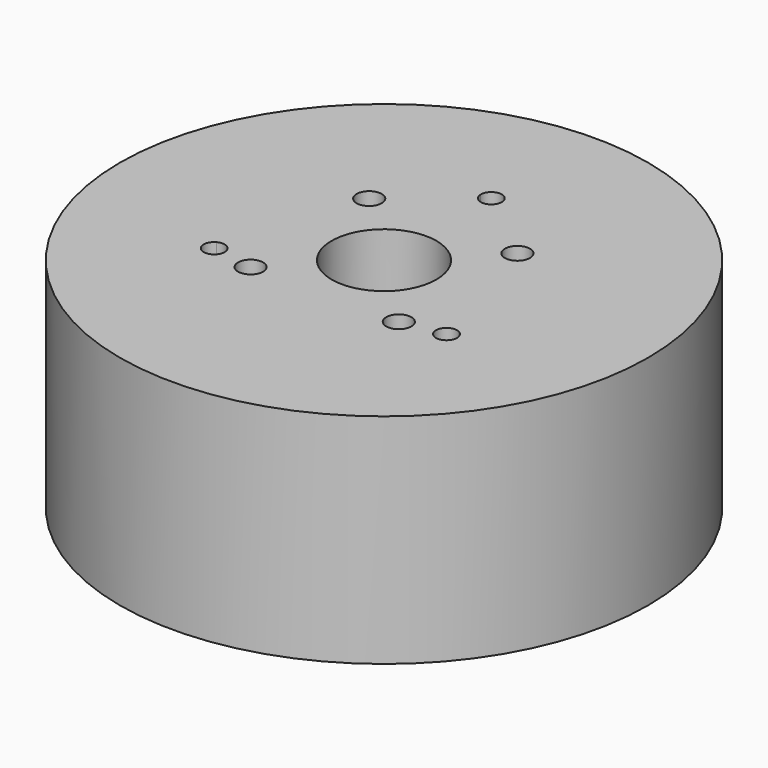
from build123d import *

# Parameters (mm, degrees)
F0_R     = 31.5
F0_R_2   = 1.5
F0_R_3   = 6.25
F1_DEPTH = 13
F2_DEPTH = 13


# Not quite as in the source:
# - a feature names something its author has since deleted; it is built from what else it names


with BuildPart() as f1:
    # F0 (on Top) → F1 (new body)
    with BuildSketch(Plane.XY):
        Circle(F0_R)
        with BuildLine():
            ThreePointArc((1.2490459616, 15.951171875), (11.7470152674, 10.8631317909), (16, 0))
            ThreePointArc((16, 0), (15.6047795357, -3.5342404619), (14.4386430447, -6.8938804043))
            ThreePointArc((14.4386430447, -6.8938804043), (14.9265222791, -7.3539720324), (15.1064064606, -8))
            ThreePointArc((15.1064064606, -8), (14.4601399606, -9.0945345408), (13.1895970831, -9.0572914707))
            ThreePointArc((13.1895970831, -9.0572914707), (0, -16), (-13.1895970831, -9.0572914707))
            ThreePointArc((-13.1895970831, -9.0572914707), (-14.9389382153, -8.625), (-14.4386430447, -6.8938804043))
            ThreePointArc((-14.4386430447, -6.8938804043), (-13.8564064606, 8), (-1.2490459616, 15.951171875))
            ThreePointArc((-1.2490459616, 15.951171875), (-0.0244187222, 17.2497614676), (1.25, 16))
            ThreePointArc((1.25, 16), (1.2497614676, 15.9755812778), (1.2490459616, 15.951171875))
        make_face(mode=Mode.SUBTRACT)
        with BuildLine():
            ThreePointArc((14.4386430447, -6.8938804043), (15.6047795357, -3.5342404619), (16, 0))
            ThreePointArc((16, 0), (11.7470152674, 10.8631317909), (1.2490459616, 15.951171875))
            ThreePointArc((1.2490459616, 15.951171875), (0, 14.75), (-1.2490459616, 15.951171875))
            ThreePointArc((-1.2490459616, 15.951171875), (-13.8564064606, 8), (-14.4386430447, -6.8938804043))
            ThreePointArc((-14.4386430447, -6.8938804043), (-13.210378493, -6.9298841815), (-12.6064064606, -8))
            ThreePointArc((-12.6064064606, -8), (-12.7618719198, -8.6037335), (-13.1895970831, -9.0572914707))
            ThreePointArc((-13.1895970831, -9.0572914707), (0, -16), (13.1895970831, -9.0572914707))
            ThreePointArc((13.1895970831, -9.0572914707), (12.7738747058, -7.375), (14.4386430447, -6.8938804043))
        make_face()
        with Locations((-8.8388347648, -8.8388347648)):
            Circle(F0_R_2, mode=Mode.SUBTRACT)
        with Locations((8.8388347648, -8.8388347648)):
            Circle(F0_R_2, mode=Mode.SUBTRACT)
        with Locations((-8.8388347648, 8.8388347648)):
            Circle(F0_R_2, mode=Mode.SUBTRACT)
        Circle(F0_R_3, mode=Mode.SUBTRACT)
        with Locations((8.8388347648, 8.8388347648)):
            Circle(F0_R_2, mode=Mode.SUBTRACT)
    extrude(amount=F1_DEPTH)

    # F0 (on Top) → F2 (join)
    with BuildSketch(Plane.XY):
        Circle(F0_R)
        with BuildLine():
            ThreePointArc((1.2490459616, 15.951171875), (11.7470152674, 10.8631317909), (16, 0))
            ThreePointArc((16, 0), (15.6047795357, -3.5342404619), (14.4386430447, -6.8938804043))
            ThreePointArc((14.4386430447, -6.8938804043), (14.9265222791, -7.3539720324), (15.1064064606, -8))
            ThreePointArc((15.1064064606, -8), (14.4601399606, -9.0945345408), (13.1895970831, -9.0572914707))
            ThreePointArc((13.1895970831, -9.0572914707), (0, -16), (-13.1895970831, -9.0572914707))
            ThreePointArc((-13.1895970831, -9.0572914707), (-14.9389382153, -8.625), (-14.4386430447, -6.8938804043))
            ThreePointArc((-14.4386430447, -6.8938804043), (-13.8564064606, 8), (-1.2490459616, 15.951171875))
            ThreePointArc((-1.2490459616, 15.951171875), (-0.0244187222, 17.2497614676), (1.25, 16))
            ThreePointArc((1.25, 16), (1.2497614676, 15.9755812778), (1.2490459616, 15.951171875))
        make_face(mode=Mode.SUBTRACT)
        with BuildLine():
            ThreePointArc((14.4386430447, -6.8938804043), (15.6047795357, -3.5342404619), (16, 0))
            ThreePointArc((16, 0), (11.7470152674, 10.8631317909), (1.2490459616, 15.951171875))
            ThreePointArc((1.2490459616, 15.951171875), (0, 14.75), (-1.2490459616, 15.951171875))
            ThreePointArc((-1.2490459616, 15.951171875), (-13.8564064606, 8), (-14.4386430447, -6.8938804043))
            ThreePointArc((-14.4386430447, -6.8938804043), (-13.210378493, -6.9298841815), (-12.6064064606, -8))
            ThreePointArc((-12.6064064606, -8), (-12.7618719198, -8.6037335), (-13.1895970831, -9.0572914707))
            ThreePointArc((-13.1895970831, -9.0572914707), (0, -16), (13.1895970831, -9.0572914707))
            ThreePointArc((13.1895970831, -9.0572914707), (12.7738747058, -7.375), (14.4386430447, -6.8938804043))
        make_face()
        with Locations((-8.8388347648, -8.8388347648)):
            Circle(F0_R_2, mode=Mode.SUBTRACT)
        with Locations((8.8388347648, -8.8388347648)):
            Circle(F0_R_2, mode=Mode.SUBTRACT)
        with Locations((-8.8388347648, 8.8388347648)):
            Circle(F0_R_2, mode=Mode.SUBTRACT)
        Circle(F0_R_3, mode=Mode.SUBTRACT)
        with Locations((8.8388347648, 8.8388347648)):
            Circle(F0_R_2, mode=Mode.SUBTRACT)
        with BuildLine():
            ThreePointArc((-1.2490459616, 15.951171875), (0, 14.75), (1.2490459616, 15.951171875))
            ThreePointArc((1.2490459616, 15.951171875), (0, 16), (-1.2490459616, 15.951171875))
        make_face()
        with BuildLine():
            ThreePointArc((-1.2490459616, 15.951171875), (0, 16), (1.2490459616, 15.951171875))
            ThreePointArc((1.2490459616, 15.951171875), (1.2497614676, 15.9755812778), (1.25, 16))
            ThreePointArc((1.25, 16), (-0.0244187222, 17.2497614676), (-1.2490459616, 15.951171875))
        make_face()
        with BuildLine():
            ThreePointArc((15.1064064606, -8), (14.9265222791, -7.3539720324), (14.4386430447, -6.8938804043))
            ThreePointArc((14.4386430447, -6.8938804043), (13.8564064606, -8), (13.1895970831, -9.0572914707))
            ThreePointArc((13.1895970831, -9.0572914707), (14.4601399606, -9.0945345408), (15.1064064606, -8))
        make_face()
        with BuildLine():
            ThreePointArc((13.1895970831, -9.0572914707), (13.8564064606, -8), (14.4386430447, -6.8938804043))
            ThreePointArc((14.4386430447, -6.8938804043), (12.7738747058, -7.375), (13.1895970831, -9.0572914707))
        make_face()
        with BuildLine():
            ThreePointArc((-12.6064064606, -8), (-13.210378493, -6.9298841815), (-14.4386430447, -6.8938804043))
            ThreePointArc((-14.4386430447, -6.8938804043), (-13.8564064606, -8), (-13.1895970831, -9.0572914707))
            ThreePointArc((-13.1895970831, -9.0572914707), (-12.7618719198, -8.6037335), (-12.6064064606, -8))
        make_face()
        with BuildLine():
            ThreePointArc((-13.1895970831, -9.0572914707), (-13.8564064606, -8), (-14.4386430447, -6.8938804043))
            ThreePointArc((-14.4386430447, -6.8938804043), (-14.9389382153, -8.625), (-13.1895970831, -9.0572914707))
        make_face()
    extrude(amount=-F2_DEPTH)


solid = f1.part
